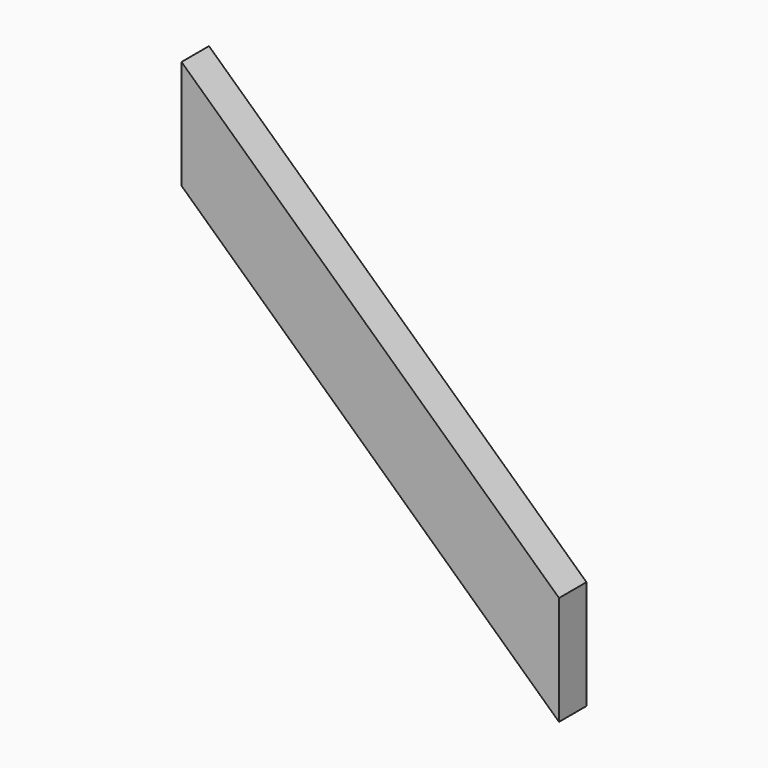
from build123d import *

# Parameters (mm, degrees)
F1_DEPTH = 38.1


# Not quite as in the source:
# - a feature names something its author has since deleted; it is built from what else it names


with BuildPart() as f1:
    # F0 (on Front) → F1 (new body)
    with BuildSketch(Plane.XZ):
        Polygon((419.0996457681, -387.6671723355), (0, 0), (0, -121.1007599326), (419.0996457681, -508.7679322681), align=None)
    extrude(amount=-F1_DEPTH)


solid = f1.part
